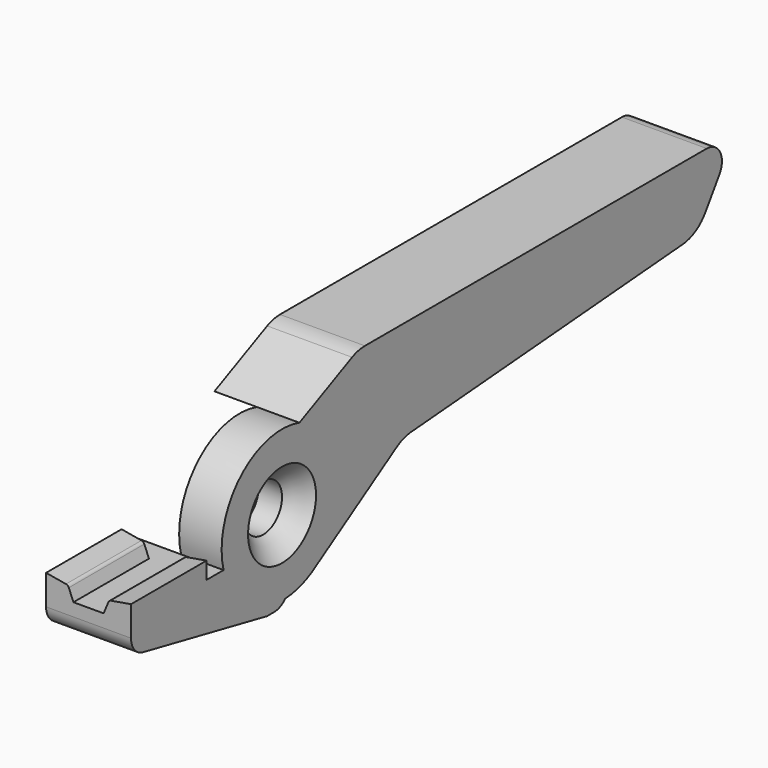
from build123d import *

# Parameters (mm, degrees)
F2_DEPTH     = 5.715
F3_R         = 5.08
F4_R         = 2.54
F0_R         = 10.16
F0_R_2       = 3.175
F5_DEPTH     = 5.715
F7_DEPTH     = 25.4
F9_DEPTH     = 5.715
F10_T1_DEPTH = 10.4031459942
F10_T3_DEPTH = 10.4031462213
F10_T5_DEPTH = 21.8251062119
F12_DEPTH    = 12.7
F13_R        = 0.508
F14_SIZE     = 2.54


# Not quite as in the source:
# - a fillet or chamfer that OpenCascade refuses, or shapes differently, is made with other operations: its cross-section is extruded or revolved along the edge and cut away or added


with BuildPart() as f2:
    # F1 (on Right) → F2 (new body, symmetric)
    with BuildSketch(Plane.YZ):
        Polygon((20.3924354673, 0.8880047341), (69.85, 4.8502287827), (76.2, 14.35636729), (12.8064267337, 14.35636729), (2.9200423986, 9.7313386741), (8.2383593544, 1.7451149179), (4.8682624474, -6.6303843632), (5.9557488763, -8.2313216024), align=None)
    extrude(amount=F2_DEPTH, both=True)

    # F3
    f3_edges = [f2.edges().sort_by_distance(p)[0] for p in [
        (0, 12.806427, 14.356367),
        (0, 69.85, 4.850229),
        (0, 20.392435, 0.888005),
    ]]
    fillet(f3_edges, radius=F3_R)

    # F4
    f4_edges = [f2.edges().sort_by_distance(p)[0] for p in [
        (0, 76.2, 14.356367),
    ]]
    fillet(f4_edges, radius=F4_R)

    # F0 (on Right) → F5 (join)
    with BuildSketch(Plane.YZ):
        Circle(F0_R)
        Circle(F0_R_2, mode=Mode.SUBTRACT)
    extrude(amount=F5_DEPTH)

    # F6 (on Right) → F7 (cut)
    with BuildSketch(Plane.YZ):
        with BuildLine():
            Line((19.0573167056, 0), (5.4165862694, 8.5957078351))
            ThreePointArc((5.4165862694, 8.5957078351), (-10.1595718617, -0.0932715764), (5.5734885208, -8.4948116935))
            Line((5.5734885208, -8.4948116935), (19.0573167056, 0))
        make_face()
    extrude(amount=-F7_DEPTH, mode=Mode.SUBTRACT)

    # F8 (on Right) → F9 (join, symmetric)
    with BuildSketch(Plane.YZ):
        with BuildLine():
            Line((0.5413664183, -10.9723807834), (0.5413664183, -10.1455666378))
            ThreePointArc((0.5413664183, -10.1455666378), (-6.0054239987, -8.1951499434), (-9.8373776994, -2.54))
            Line((-9.8373776994, -2.54), (-25.4, -2.54))
            Line((-25.4, -2.54), (-25.4, -6.360667292))
            Line((-25.4, -6.360667292), (-2.5253696451, -10.9723807834))
            Line((-2.5253696451, -10.9723807834), (0.5413664183, -10.9723807834))
        make_face()
    extrude(amount=F9_DEPTH, both=True)

    # F10: fillet of radius 2.54 on 2 edges, made by hand

    # F10_s2 → F10_t1 (cut)
    with BuildSketch(Plane.YZ.offset(-10.4031461077)):
        with BuildLine():
            ThreePointArc((0.5413664183, -10.1455666378), (-0.3091706163, -10.7565034211), (-1.3338920247, -10.9723807834))
            Line((-1.3338920247, -10.9723807834), (0.5413664183, -10.9723807834))
            Line((0.5413664183, -10.9723807834), (0.5413664183, -10.1455666378))
        make_face()
    extrude(amount=F10_T1_DEPTH, mode=Mode.SUBTRACT)

    # F10_s4 → F10_t3 (cut)
    with BuildSketch(Plane.YZ.offset(-1.135e-07)):
        with BuildLine():
            ThreePointArc((0.5413664183, -10.1455666378), (-0.3091706163, -10.7565034211), (-1.3338920247, -10.9723807834))
            Line((-1.3338920247, -10.9723807834), (0.5413664183, -10.9723807834))
            Line((0.5413664183, -10.9723807834), (0.5413664183, -10.1455666378))
        make_face()
    extrude(amount=F10_T3_DEPTH, mode=Mode.SUBTRACT)

    # F10_s6 → F10_t5 (cut)
    with BuildSketch(Plane.YZ.offset(-10.912553106)):
        with BuildLine():
            ThreePointArc((-25.4, -4.2816460496), (-24.8255331463, -5.8904591062), (-23.3619846843, -6.7715479306))
            Line((-23.3619846843, -6.7715479306), (-25.4, -6.360667292))
            Line((-25.4, -6.360667292), (-25.4, -4.2816460496))
        make_face()
    extrude(amount=F10_T5_DEPTH, mode=Mode.SUBTRACT)

    # F11 (on face) → F12 (join)
    with BuildSketch(Plane.XZ.offset(25.4)):
        Polygon((2.7630305849, -0.762), (2.032, -2.54), (5.715, -2.54), (5.715, -0.254), align=None)
        Polygon((-5.715, -2.54), (-2.032, -2.54), (-2.7630305849, -0.762), (-5.715, -0.254), align=None)
    extrude(amount=-F12_DEPTH)

    # F13
    f13_edges = [f2.edges().sort_by_distance(p)[0] for p in [
        (-2.763031, -19.05, -0.762),
        (2.763031, -19.05, -0.762),
    ]]
    fillet(f13_edges, radius=F13_R)

    # F14
    f14_edges = [f2.edges().sort_by_distance(p)[0] for p in [
        (5.715, -3.175, 0),
    ]]
    chamfer(f14_edges, length=F14_SIZE)


solid = f2.part
